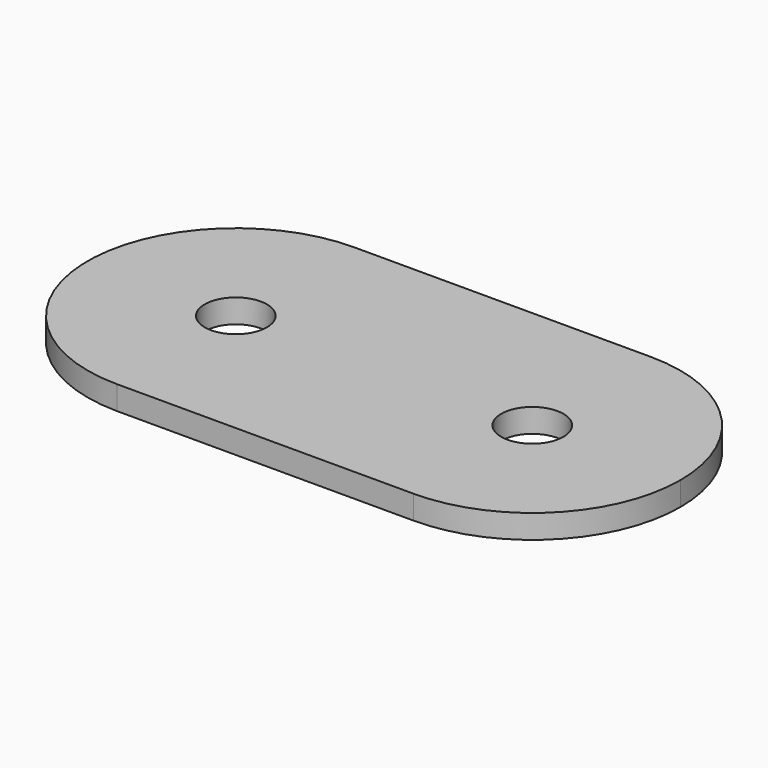
from build123d import *

# Parameters (mm, degrees)
F0_R     = 2.1
F1_DEPTH = 1.6


# Not quite as in the source:
# - a feature names something its author has since deleted; it is built from what else it names


with BuildPart() as f1:
    # F0 (on Top) → F1 (new body)
    with BuildSketch(Plane.XY):
        with BuildLine():
            ThreePointArc((-10, -10), (-2.9289321881, -7.0710678119), (0, 0))
            ThreePointArc((0, 0), (-2.9289321881, 7.0710678119), (-10, 10))
            ThreePointArc((-10, 10), (-20, 0), (-10, -10))
        make_face()
        with Locations((-10, 0)):
            Circle(F0_R, mode=Mode.SUBTRACT)
        with BuildLine():
            ThreePointArc((10, 10), (2.9289321881, 7.0710678119), (0, 0))
            ThreePointArc((0, 0), (2.9289321881, -7.0710678119), (10, -10))
            ThreePointArc((10, -10), (17.0710678119, -7.0710678119), (20, 0))
            ThreePointArc((20, 0), (17.0710678119, 7.0710678119), (10, 10))
        make_face()
        with Locations((10, 0)):
            Circle(F0_R, mode=Mode.SUBTRACT)
        with BuildLine():
            ThreePointArc((-10, 10), (-2.9289321881, 7.0710678119), (0, 0))
            ThreePointArc((0, 0), (2.9289321881, 7.0710678119), (10, 10))
            Line((10, 10), (-10, 10))
        make_face()
        with BuildLine():
            ThreePointArc((10, -10), (2.9289321881, -7.0710678119), (0, 0))
            ThreePointArc((0, 0), (-2.9289321881, -7.0710678119), (-10, -10))
            Line((-10, -10), (10, -10))
        make_face()
    extrude(amount=F1_DEPTH)


solid = f1.part
